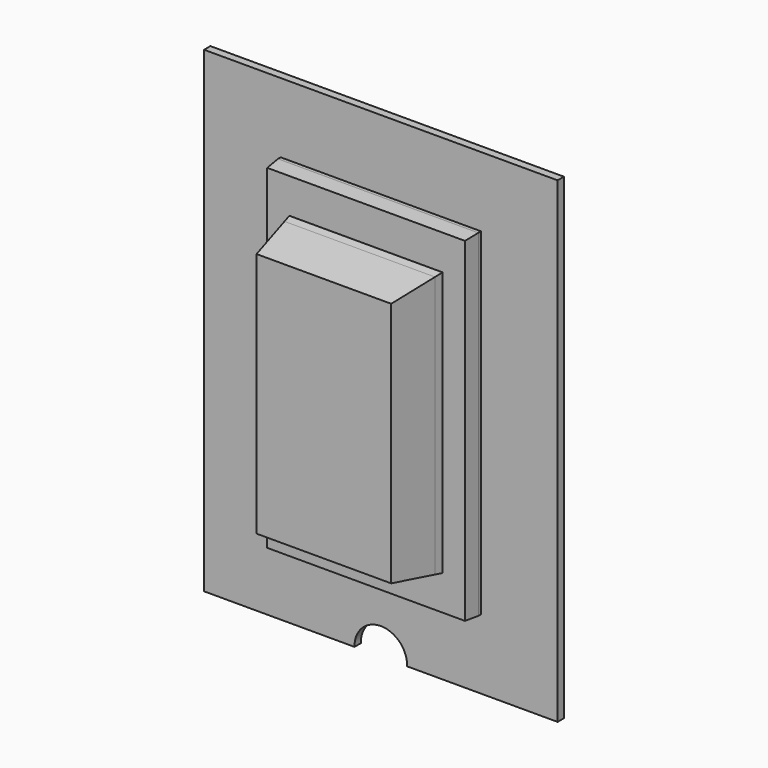
from build123d import *

# Parameters (mm, degrees)
F0_W         = 57.0548474789
F0_H         = 99.3303954601
F1_DEPTH     = 30
F0_W_2       = 75.9585499763
F0_H_2       = 127.8578191996
F2_DEPTH     = 10
F3_C1_SIZE2  = 3
F3_C1_SIZE   = 17.0138454589
F3_C2_SIZE2  = 3
F3_C2_SIZE   = 17.0138454589
F3_C3_SIZE2  = 3
F3_C3_SIZE   = 17.0138454589
F3_C4_SIZE2  = 3
F3_C4_SIZE   = 17.0138454589
F4_T4_DEPTH  = 57.0548474789
F4_T9_DEPTH  = 99.3303954601
F4_T14_DEPTH = 57.0548474789
F4_T19_DEPTH = 99.3303954601
F4_T25_DEPTH = 114.1873722104
F4_T31_DEPTH = 71.9118242292
F4_T40_DEPTH = 114.1873722104
F4_T46_DEPTH = 71.9118242292
F4_T55_DEPTH = 71.9118242292
F4_T61_DEPTH = 114.1873722104
F4_T70_DEPTH = 71.9118242292
F4_T76_DEPTH = 114.1873722104
F4_T81_DEPTH = 157.5717727001
F4_T83_DEPTH = 105.6725034769
F0_W_3       = 134.0444982052
F0_H_3       = 180.7882040739
F5_DEPTH     = 3
F7_D         = 20


# Not quite as in the source:
# - a fillet or chamfer that OpenCascade refuses, or shapes differently, is made with other operations: its cross-section is extruded or revolved along the edge and cut away or added


with BuildPart() as f1:
    # F0 (on Front) → F1 (new body)
    with BuildSketch(Plane.XZ):
        Rectangle(F0_W, F0_H)
    extrude(amount=F1_DEPTH)

    # F0 (on Front) → F2 (join)
    with BuildSketch(Plane.XZ):
        Rectangle(F0_W_2, F0_H_2)
        Rectangle(F0_W, F0_H, mode=Mode.SUBTRACT)
    extrude(amount=F2_DEPTH)

    # F3: chamfer of 3 x 17.0138454589 on 4 edges, made by hand

    # F3_c1
    f3_c1_edges = [f1.edges().sort_by_distance(p)[0] for p in [
        (28.5274237394, -30, 0),
    ]]
    f3_c1_side = f1.faces().sort_by_distance((28.5274237394, -29.94, 0))[0]
    chamfer(f3_c1_edges, length=F3_C1_SIZE, length2=F3_C1_SIZE2, reference=f3_c1_side)

    # F3_c2
    f3_c2_edges = [f1.edges().sort_by_distance(p)[0] for p in [
        (-1.5, -30, 49.6651977301),
    ]]
    f3_c2_side = f1.faces().sort_by_distance((-1.5, -29.94, 49.6651977301))[0]
    chamfer(f3_c2_edges, length=F3_C2_SIZE, length2=F3_C2_SIZE2, reference=f3_c2_side)

    # F3_c3
    f3_c3_edges = [f1.edges().sort_by_distance(p)[0] for p in [
        (-28.5274237394, -30, -1.5),
    ]]
    f3_c3_side = f1.faces().sort_by_distance((-28.5274237394, -29.94, -1.5))[0]
    chamfer(f3_c3_edges, length=F3_C3_SIZE, length2=F3_C3_SIZE2, reference=f3_c3_side)

    # F3_c4
    f3_c4_edges = [f1.edges().sort_by_distance(p)[0] for p in [
        (0, -30, -49.6651977301),
    ]]
    f3_c4_side = f1.faces().sort_by_distance((0, -29.94, -49.6651977301))[0]
    chamfer(f3_c4_edges, length=F3_C4_SIZE, length2=F3_C4_SIZE2, reference=f3_c4_side)

    # F4: chamfer of 0.5 x 5.7150261514 on 8 edges, made by hand


with BuildPart() as f4_tool2:
    # F4_s3 → F4_t4 (new body)
    with BuildSketch(Plane.YZ.offset(-28.5274237394)):
        Polygon((-10, 50.1651977301), (-15.7150261514, 49.6651977301), (-10, 49.6651977301), align=None)
    extrude(amount=F4_T4_DEPTH)

    split(bisect_by=Plane(origin=(0, -8.8848294962, 50.3883719921), x_dir=(1, 0, 0), z_dir=(0, 0.1736481777, -0.984807753)), keep=Keep.TOP)


with BuildPart() as f1_1:
    add(f1.part)

    # F4_t1: union F4_tool2
    add(f4_tool2.part)


with BuildPart() as f4_tool7:
    # F4_s8 → F4_t9 (new body)
    with BuildSketch(Plane.XY.offset(49.6651977301)):
        Polygon((28.5274237394, -15.7150261514), (29.0274237394, -10), (28.5274237394, -10), align=None)
    extrude(amount=-F4_T9_DEPTH)

    split(bisect_by=Plane(origin=(29.8879798774, -5.2700572513, 0), x_dir=(0, 0, 1), z_dir=(-0.984807753, 0.1736481777, 0)), keep=Keep.TOP)


with BuildPart() as f1_2:
    add(f1_1.part)

    # F4_t6: union F4_tool7
    add(f4_tool7.part)


with BuildPart() as f4_tool12:
    # F4_s13 → F4_t14 (new body)
    with BuildSketch(Plane.YZ.offset(28.5274237394)):
        Polygon((-15.7150261514, -49.6651977301), (-10, -50.1651977301), (-10, -49.6651977301), align=None)
    extrude(amount=-F4_T14_DEPTH)

    split(bisect_by=Plane(origin=(0, -8.8848294962, -50.3883719921), x_dir=(1, 0, 0), z_dir=(0, 0.1736481777, 0.984807753)), keep=Keep.TOP)


with BuildPart() as f1_3:
    add(f1_2.part)

    # F4_t11: union F4_tool12
    add(f4_tool12.part)


with BuildPart() as f4_tool17:
    # F4_s18 → F4_t19 (new body)
    with BuildSketch(Plane.XY.offset(-49.6651977301)):
        Polygon((-28.5274237394, -15.7150261514), (-29.0274237394, -10), (-28.5274237394, -10), align=None)
    extrude(amount=F4_T19_DEPTH)

    split(bisect_by=Plane(origin=(-29.8879798774, -5.2700572513, 0), x_dir=(0, 0, 1), z_dir=(0.984807753, 0.1736481777, 0)), keep=Keep.TOP)


with BuildPart() as f1_4:
    add(f1_3.part)

    # F4_t16: union F4_tool17
    add(f4_tool17.part)


with BuildPart() as f4_tool23:
    # F4_s24 → F4_t25 (new body)
    with BuildSketch(Plane.XY.offset(-49.6651977301)):
        Polygon((-28.5274237394, -15.7150261514), (-29.0274237394, -10), (-28.5274237394, -10), align=None)
    extrude(amount=F4_T25_DEPTH)

    split(bisect_by=Plane(origin=(-29.8879798774, -5.2700572513, 0), x_dir=(0, 0, 1), z_dir=(0.984807753, 0.1736481777, 0)), keep=Keep.TOP)

    split(bisect_by=Plane.XY.offset(49.6651977301), keep=Keep.TOP)

    split(bisect_by=Plane.XY.offset(63.9289095998), keep=Keep.BOTTOM)


with BuildPart() as f4_tool29:
    # F4_s30 → F4_t31 (new body)
    with BuildSketch(Plane.YZ.offset(-43.3844004897)):
        Polygon((-10, 50.1651977301), (-15.7150261514, 49.6651977301), (-10, 49.6651977301), align=None)
    extrude(amount=F4_T31_DEPTH)

    split(bisect_by=Plane.YZ.offset(-28.5274237394), keep=Keep.BOTTOM)

    split(bisect_by=Plane.YZ.offset(-37.9792749882), keep=Keep.TOP)

    split(bisect_by=Plane(origin=(0, -8.8848294962, 50.3883719921), x_dir=(1, 0, 0), z_dir=(0, 0.1736481777, -0.984807753)), keep=Keep.TOP)


with BuildPart() as f4_tool23_1:
    add(f4_tool23.part)

    # F4_t35: intersect F4_tool29
    add(f4_tool29.part, mode=Mode.INTERSECT)


with BuildPart() as f1_5:
    add(f1_4.part)

    # F4_t21: union F4_tool23
    add(f4_tool23_1.part)


with BuildPart() as f4_tool38:
    # F4_s39 → F4_t40 (new body)
    with BuildSketch(Plane.XY.offset(64.5221744803)):
        Polygon((28.5274237394, -15.7150261514), (29.0274237394, -10), (28.5274237394, -10), align=None)
    extrude(amount=-F4_T40_DEPTH)

    split(bisect_by=Plane.XY.offset(49.6651977301), keep=Keep.TOP)

    split(bisect_by=Plane(origin=(29.8879798774, -5.2700572513, 0), x_dir=(0, 0, 1), z_dir=(-0.984807753, 0.1736481777, 0)), keep=Keep.TOP)

    split(bisect_by=Plane.XY.offset(63.9289095998), keep=Keep.BOTTOM)


with BuildPart() as f4_tool44:
    # F4_s45 → F4_t46 (new body)
    with BuildSketch(Plane.YZ.offset(-28.5274237394)):
        Polygon((-10, 50.1651977301), (-15.7150261514, 49.6651977301), (-10, 49.6651977301), align=None)
    extrude(amount=F4_T46_DEPTH)

    split(bisect_by=Plane.YZ.offset(28.5274237394), keep=Keep.TOP)

    split(bisect_by=Plane.YZ.offset(37.9792749882), keep=Keep.BOTTOM)

    split(bisect_by=Plane(origin=(0, -8.8848294962, 50.3883719921), x_dir=(1, 0, 0), z_dir=(0, 0.1736481777, -0.984807753)), keep=Keep.TOP)


with BuildPart() as f4_tool38_1:
    add(f4_tool38.part)

    # F4_t50: intersect F4_tool44
    add(f4_tool44.part, mode=Mode.INTERSECT)


with BuildPart() as f1_6:
    add(f1_5.part)

    # F4_t36: union F4_tool38
    add(f4_tool38_1.part)


with BuildPart() as f4_tool53:
    # F4_s54 → F4_t55 (new body)
    with BuildSketch(Plane.YZ.offset(43.3844004897)):
        Polygon((-15.7150261514, -49.6651977301), (-10, -50.1651977301), (-10, -49.6651977301), align=None)
    extrude(amount=-F4_T55_DEPTH)

    split(bisect_by=Plane(origin=(0, -8.8848294962, -50.3883719921), x_dir=(1, 0, 0), z_dir=(0, 0.1736481777, 0.984807753)), keep=Keep.TOP)

    split(bisect_by=Plane.YZ.offset(28.5274237394), keep=Keep.TOP)

    split(bisect_by=Plane.YZ.offset(37.9792749882), keep=Keep.BOTTOM)


with BuildPart() as f4_tool59:
    # F4_s60 → F4_t61 (new body)
    with BuildSketch(Plane.XY.offset(49.6651977301)):
        Polygon((28.5274237394, -15.7150261514), (29.0274237394, -10), (28.5274237394, -10), align=None)
    extrude(amount=-F4_T61_DEPTH)

    split(bisect_by=Plane.XY.offset(-49.6651977301), keep=Keep.BOTTOM)

    split(bisect_by=Plane(origin=(29.8879798774, -5.2700572513, 0), x_dir=(0, 0, 1), z_dir=(-0.984807753, 0.1736481777, 0)), keep=Keep.TOP)

    split(bisect_by=Plane.XY.offset(-63.9289095998), keep=Keep.TOP)


with BuildPart() as f4_tool53_1:
    add(f4_tool53.part)

    # F4_t65: intersect F4_tool59
    add(f4_tool59.part, mode=Mode.INTERSECT)


with BuildPart() as f1_7:
    add(f1_6.part)

    # F4_t51: union F4_tool53
    add(f4_tool53_1.part)


with BuildPart() as f4_tool68:
    # F4_s69 → F4_t70 (new body)
    with BuildSketch(Plane.YZ.offset(28.5274237394)):
        Polygon((-15.7150261514, -49.6651977301), (-10, -50.1651977301), (-10, -49.6651977301), align=None)
    extrude(amount=-F4_T70_DEPTH)

    split(bisect_by=Plane(origin=(0, -8.8848294962, -50.3883719921), x_dir=(1, 0, 0), z_dir=(0, 0.1736481777, 0.984807753)), keep=Keep.TOP)

    split(bisect_by=Plane.YZ.offset(-28.5274237394), keep=Keep.BOTTOM)

    split(bisect_by=Plane.YZ.offset(-37.9792749882), keep=Keep.TOP)


with BuildPart() as f4_tool74:
    # F4_s75 → F4_t76 (new body)
    with BuildSketch(Plane.XY.offset(-64.5221744803)):
        Polygon((-28.5274237394, -15.7150261514), (-29.0274237394, -10), (-28.5274237394, -10), align=None)
    extrude(amount=F4_T76_DEPTH)

    split(bisect_by=Plane.XY.offset(-49.6651977301), keep=Keep.BOTTOM)

    split(bisect_by=Plane(origin=(-29.8879798774, -5.2700572513, 0), x_dir=(0, 0, 1), z_dir=(0.984807753, 0.1736481777, 0)), keep=Keep.TOP)

    split(bisect_by=Plane.XY.offset(-63.9289095998), keep=Keep.TOP)


with BuildPart() as f4_tool68_1:
    add(f4_tool68.part)

    # F4_t80: intersect F4_tool74
    add(f4_tool74.part, mode=Mode.INTERSECT)


with BuildPart() as f1_8:
    add(f1_7.part)

    # F4_t66: union F4_tool68
    add(f4_tool68_1.part)

    # F4_s82 → F4_t81 (cut)
    with BuildSketch(Plane.XY.offset(-78.7858863501)):
        Polygon((37.4792749882, -10), (37.9792749882, -4.2849738486), (37.9792749882, -10), align=None)
        Polygon((-37.4792749882, -10), (-37.9792749882, -4.2849738486), (-37.9792749882, -10), align=None)
    extrude(amount=F4_T81_DEPTH, mode=Mode.SUBTRACT)

    # F4_s84 → F4_t83 (cut)
    with BuildSketch(Plane.YZ.offset(-52.8362517385)):
        Polygon((-10, 63.4289095998), (-4.2849738486, 63.9289095998), (-10, 63.9289095998), align=None)
        Polygon((-10, -63.4289095998), (-4.2849738486, -63.9289095998), (-10, -63.9289095998), align=None)
    extrude(amount=F4_T83_DEPTH, mode=Mode.SUBTRACT)

    # F0 (on Front) → F5 (join)
    with BuildSketch(Plane.XZ):
        Rectangle(F0_W_3, F0_H_3)
        Rectangle(F0_W_2, F0_H_2, mode=Mode.SUBTRACT)
    extrude(amount=F5_DEPTH)

    # F7 (through all)
    with Locations(Plane(origin=(0, 0, 0), x_dir=(1, 0, 0), z_dir=(0, 1, 0))):
        with Locations((0, 90.1845097542)):
            Hole(F7_D / 2)


solid = f1_8.part
